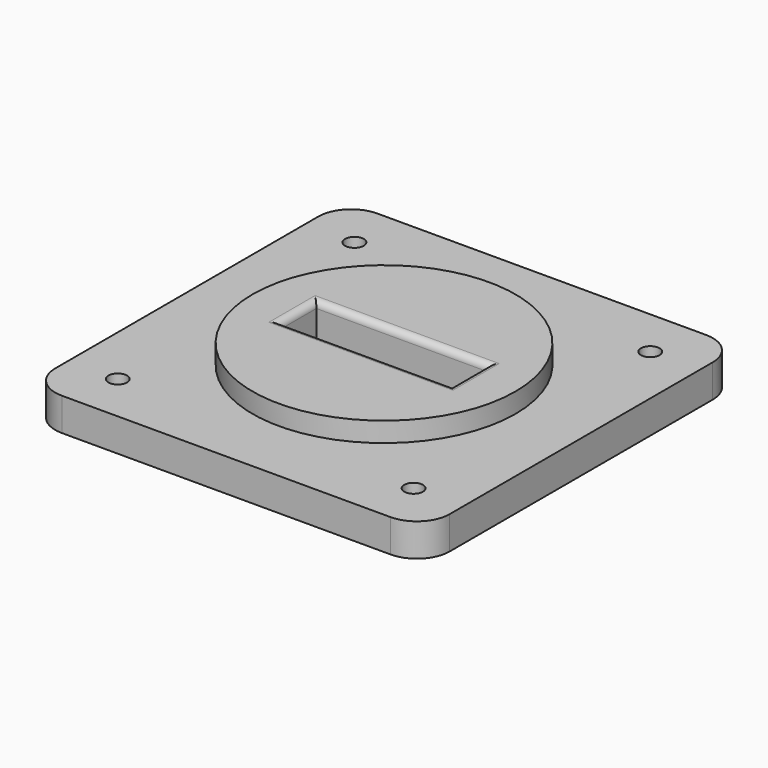
from build123d import *

# Parameters (mm, degrees)
F0_R     = 1.8034
F0_R_2   = 25.4
F0_W     = 33.02
F0_H     = 8.636
F1_DEPTH = 6.35
F2_R     = 25.4
F3_DEPTH = 3.81
F4_DEPTH = 12.7
F5_R     = 1.27


# Not quite as in the source:
# - a feature names something its author has since deleted; it is built from what else it names


with BuildPart() as f1:
    # F0 (on Top) → F1 (new body)
    with BuildSketch(Plane.XY):
        with BuildLine():
            Line((-31.75, -38.1), (31.75, -38.1))
            ThreePointArc((31.75, -38.1), (36.2401280605, -36.2401280605), (38.1, -31.75))
            Line((38.1, -31.75), (38.1, 31.75))
            ThreePointArc((38.1, 31.75), (36.2401280605, 36.2401280605), (31.75, 38.1))
            Line((31.75, 38.1), (-31.75, 38.1))
            ThreePointArc((-31.75, 38.1), (-36.2401280605, 36.2401280605), (-38.1, 31.75))
            Line((-38.1, 31.75), (-38.1, -31.75))
            ThreePointArc((-38.1, -31.75), (-36.2401280605, -36.2401280605), (-31.75, -38.1))
        make_face()
        with Locations((-28.575, -28.575)):
            Circle(F0_R, mode=Mode.SUBTRACT)
        with Locations((28.575, -28.575)):
            Circle(F0_R, mode=Mode.SUBTRACT)
        with Locations((-28.575, 28.575)):
            Circle(F0_R, mode=Mode.SUBTRACT)
        Circle(F0_R_2, mode=Mode.SUBTRACT)
        with Locations((28.575, 28.575)):
            Circle(F0_R, mode=Mode.SUBTRACT)
        Circle(F0_R_2)
        with Locations((0, -8.382)):
            Circle(F0_R, mode=Mode.SUBTRACT)
        Rectangle(F0_W, F0_H, mode=Mode.SUBTRACT)
        with Locations((0, 8.382)):
            Circle(F0_R, mode=Mode.SUBTRACT)
    extrude(amount=F1_DEPTH)

    # F2 (on face) → F3 (join)
    with BuildSketch(Plane.XY.offset(6.35)):
        Circle(F2_R)
    extrude(amount=F3_DEPTH)

    # F0 (on Top) → F4 (cut, symmetric)
    with BuildSketch(Plane.XY):
        Rectangle(F0_W, F0_H)
    extrude(amount=F4_DEPTH, both=True, mode=Mode.SUBTRACT)

    # F5
    f5_edges = [f1.edges().sort_by_distance(p)[0] for p in [
        (0, 4.318, 10.16),
        (-16.51, 0, 10.16),
        (0, -4.318, 10.16),
        (16.51, 0, 10.16),
    ]]
    fillet(f5_edges, radius=F5_R)


solid = f1.part
